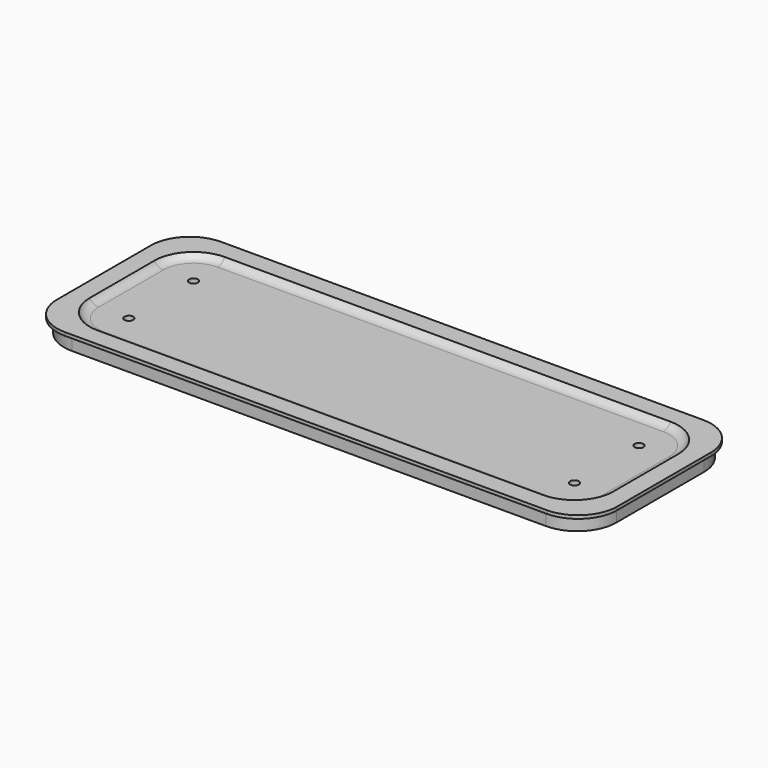
from build123d import *

# Parameters (mm, degrees)
F0_W          = 215
F0_H          = 75
F1_DEPTH      = 1.25
F2_R          = 15
F3_W          = 212
F3_H          = 72
F4_DEPTH      = 5.25
F5_T1_DEPTH   = 42.75
F7_W          = 201
F7_H          = 61
F8_DEPTH      = 2
F9_R          = 15
F10_T1_DEPTH  = 31
F10_T3_DEPTH  = 171
F10_T6_ANGLE  = 90
F10_T8_ANGLE  = 90
F10_T10_ANGLE = 90
F10_T12_ANGLE = 90
F11_W         = 45.625
F11_H         = 3.75
F12_DEPTH     = 12
F13_W         = 153
F13_H         = 55
F14_DEPTH     = 4
F16_D         = 3.4


# Not quite as in the source:
# - a fillet or chamfer that OpenCascade refuses, or shapes differently, is made with other operations: its cross-section is extruded or revolved along the edge and cut away or added


with BuildPart() as f1:
    # F0 (on Top) → F1 (new body)
    with BuildSketch(Plane.XY):
        Rectangle(F0_W, F0_H)
    extrude(amount=F1_DEPTH)

    # F2
    f2_edges = [f1.edges().sort_by_distance(p)[0] for p in [
        (107.5, -37.5, 0.625),
        (107.5, 37.5, 0.625),
        (-107.5, 37.5, 0.625),
        (-107.5, -37.5, 0.625),
    ]]
    fillet(f2_edges, radius=F2_R)

    # F3 (on face) → F4 (join)
    with BuildSketch(Plane(origin=(0, 0, 0), x_dir=(1, 0, 0), z_dir=(0, 0, -1))):
        Rectangle(F3_W, F3_H)
    extrude(amount=F4_DEPTH)

    # F5: fillet of radius 15 on 4 edges, made by hand

    # F5_s2 → F5_t1 (cut)
    with BuildSketch(Plane.XY.offset(-42.75)):
        with BuildLine():
            ThreePointArc((-106, -21), (-101.6066017178, -31.6066017178), (-91, -36))
            Line((-91, -36), (-106, -36))
            Line((-106, -36), (-106, -21))
        make_face()
        with BuildLine():
            ThreePointArc((-91, 36), (-101.6066017178, 31.6066017178), (-106, 21))
            Line((-106, 21), (-106, 36))
            Line((-106, 36), (-91, 36))
        make_face()
        with BuildLine():
            ThreePointArc((91, 36), (101.6066017178, 31.6066017178), (106, 21))
            Line((106, 21), (106, 36))
            Line((106, 36), (91, 36))
        make_face()
        with BuildLine():
            ThreePointArc((106, -21), (101.6066017178, -31.6066017178), (91, -36))
            Line((91, -36), (106, -36))
            Line((106, -36), (106, -21))
        make_face()
    extrude(amount=F5_T1_DEPTH, mode=Mode.SUBTRACT)

    # F7 (on face) → F8 (cut)
    with BuildSketch(Plane.XY.offset(1.25)):
        Rectangle(F7_W, F7_H)
    extrude(amount=-F8_DEPTH, mode=Mode.SUBTRACT)

    # F9
    f9_edges = [f1.edges().sort_by_distance(p)[0] for p in [
        (-100.5, 30.5, 0.25),
        (-100.5, -30.5, 0.25),
        (100.5, 30.5, 0.25),
        (100.5, -30.5, 0.25),
    ]]
    fillet(f9_edges, radius=F9_R)

    # F10: fillet of radius 4 on 1 edges, made by hand

    # F10_s2 → F10_t1 (join)
    with BuildSketch(Plane.XZ.offset(-15.5)):
        with BuildLine():
            ThreePointArc((-100.5, 1.25), (-99.0358983849, -0.2141016151), (-97.0358983849, -0.75))
            Line((-97.0358983849, -0.75), (-100.5, -0.75))
            Line((-100.5, -0.75), (-100.5, 1.25))
        make_face()
        with BuildLine():
            ThreePointArc((100.5, 1.25), (99.0358983849, -0.2141016151), (97.0358983849, -0.75))
            Line((97.0358983849, -0.75), (100.5, -0.75))
            Line((100.5, -0.75), (100.5, 1.25))
        make_face()
    extrude(amount=F10_T1_DEPTH)

    # F10_s4 → F10_t3 (join)
    with BuildSketch(Plane.YZ.offset(-85.5)):
        with BuildLine():
            ThreePointArc((-30.5, 1.25), (-29.0358983849, -0.2141016151), (-27.0358983849, -0.75))
            Line((-27.0358983849, -0.75), (-30.5, -0.75))
            Line((-30.5, -0.75), (-30.5, 1.25))
        make_face()
        with BuildLine():
            ThreePointArc((30.5, 1.25), (29.0358983849, -0.2141016151), (27.0358983849, -0.75))
            Line((27.0358983849, -0.75), (30.5, -0.75))
            Line((30.5, -0.75), (30.5, 1.25))
        make_face()
    extrude(amount=F10_T3_DEPTH)

    # F10_s5 → F10_t6 (revolve)
    with BuildSketch(Plane.YZ.offset(-85.5)):
        with BuildLine():
            ThreePointArc((30.5, 1.25), (29.0358983849, -0.2141016151), (27.0358983849, -0.75))
            Line((27.0358983849, -0.75), (30.5, -0.75))
            Line((30.5, -0.75), (30.5, 1.25))
        make_face()
    revolve(axis=Axis((-85.5, 15.5, -0.75), (0, 0, 1)), revolution_arc=F10_T6_ANGLE)

    # F10_s7 → F10_t8 (revolve)
    with BuildSketch(Plane.XZ.offset(15.5)):
        with BuildLine():
            ThreePointArc((-100.5, 1.25), (-99.0358983849, -0.2141016151), (-97.0358983849, -0.75))
            Line((-97.0358983849, -0.75), (-100.5, -0.75))
            Line((-100.5, -0.75), (-100.5, 1.25))
        make_face()
    revolve(axis=Axis((-85.5, -15.5, -0.75), (0, 0, 1)), revolution_arc=F10_T8_ANGLE)

    # F10_s9 → F10_t10 (revolve)
    with BuildSketch(Plane.YZ.offset(85.5)):
        with BuildLine():
            ThreePointArc((-30.5, 1.25), (-29.0358983849, -0.2141016151), (-27.0358983849, -0.75))
            Line((-27.0358983849, -0.75), (-30.5, -0.75))
            Line((-30.5, -0.75), (-30.5, 1.25))
        make_face()
    revolve(axis=Axis((85.5, -15.5, -0.75), (0, 0, 1)), revolution_arc=F10_T10_ANGLE)

    # F10_s11 → F10_t12 (revolve)
    with BuildSketch(Plane.YZ.offset(85.5)):
        with BuildLine():
            ThreePointArc((30.5, 1.25), (29.0358983849, -0.2141016151), (27.0358983849, -0.75))
            Line((27.0358983849, -0.75), (30.5, -0.75))
            Line((30.5, -0.75), (30.5, 1.25))
        make_face()
    revolve(axis=Axis((85.5, 15.5, -0.75), (0, 0, -1)), revolution_arc=F10_T12_ANGLE)

    # F11 (on face) → F12 (cut)
    with BuildSketch(Plane(origin=(0, 36, 0), x_dir=(-1, 0, 0), z_dir=(0, 1, 0))):
        with Locations((-53.6875, -3.375)):
            Rectangle(F11_W, F11_H)
        with Locations((53.6875, -3.375)):
            Rectangle(F11_W, F11_H)
    extrude(amount=-F12_DEPTH, mode=Mode.SUBTRACT)

    # F13 (on face) → F14 (cut)
    with BuildSketch(Plane(origin=(0, 0, -5.25), x_dir=(1, 0, 0), z_dir=(0, 0, -1))):
        with Locations((0, 6)):
            Rectangle(F13_W, F13_H)
    extrude(amount=-F14_DEPTH, mode=Mode.SUBTRACT)

    # F16 (through all)
    with Locations(Plane.XY.offset(1.25)):
        with Locations((-85.5, 15.5), (-85.5, -15.5), (85.5, 15.5), (85.5, -15.5)):
            Hole(F16_D / 2)


solid = f1.part
